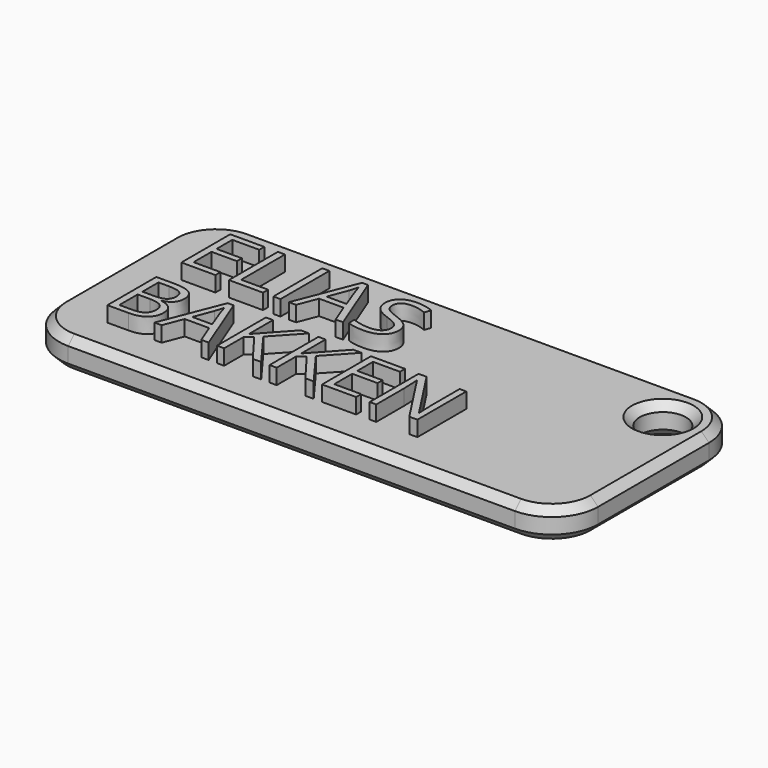
from build123d import *

# Parameters (mm, degrees)
F0_W         = 35
F0_H         = 15
F0_R         = 1.5
F1_DEPTH     = 2
F2_R         = 3
F3_TEXT_SIZE = 5.5555555556
F4_DEPTH     = 1
F5_SIZE      = 0.5
F6_SIZE      = 0.5


# Not quite as in the source:
# - Text() gives the source's letters only with a copy of the font that has no kerning and outlines rounded to 1/6400 em; it was checked with that copy


with BuildPart() as f1:
    # F0 (on Top) → F1 (new body)
    with BuildSketch(Plane.XY):
        Rectangle(F0_W, F0_H)
        with Locations((14.5, 4.5)):
            Circle(F0_R, mode=Mode.SUBTRACT)
    extrude(amount=F1_DEPTH)

    # F2
    f2_edges = [f1.edges().sort_by_distance(p)[0] for p in [
        (-17.5, 7.5, 1),
        (-17.5, -7.5, 1),
        (17.5, -7.5, 1),
        (17.5, 7.5, 1),
    ]]
    fillet(f2_edges, radius=F2_R)

    # F3 (on face) → F4 (join)
    with BuildSketch(Plane.XY.offset(2)):
        with Locations((-14.5, 1)):
            Text('ELIAS', F3_TEXT_SIZE, font='Open Sans', text_align=(TextAlign.LEFT, TextAlign.BOTTOM))
        with Locations((-14.5, -5)):
            Text('BAKKEN', F3_TEXT_SIZE, font='Open Sans', text_align=(TextAlign.LEFT, TextAlign.BOTTOM))
    extrude(amount=F4_DEPTH)

    # F5
    f5_edges = [f1.edges().sort_by_distance(p)[0] for p in [
        (16, 4.5, 1),
        (13, 4.5, 0),
        (13, 4.5, 2),
    ]]
    chamfer(f5_edges, length=F5_SIZE)

    # F6
    f6_edges = [f1.edges().sort_by_distance(p)[0] for p in [
        (0, 7.5, 0),
        (14.5, 7.5, 1),
        (-14.5, 7.5, 1),
        (0, 7.5, 2),
    ]]
    chamfer(f6_edges, length=F6_SIZE)


solid = f1.part
